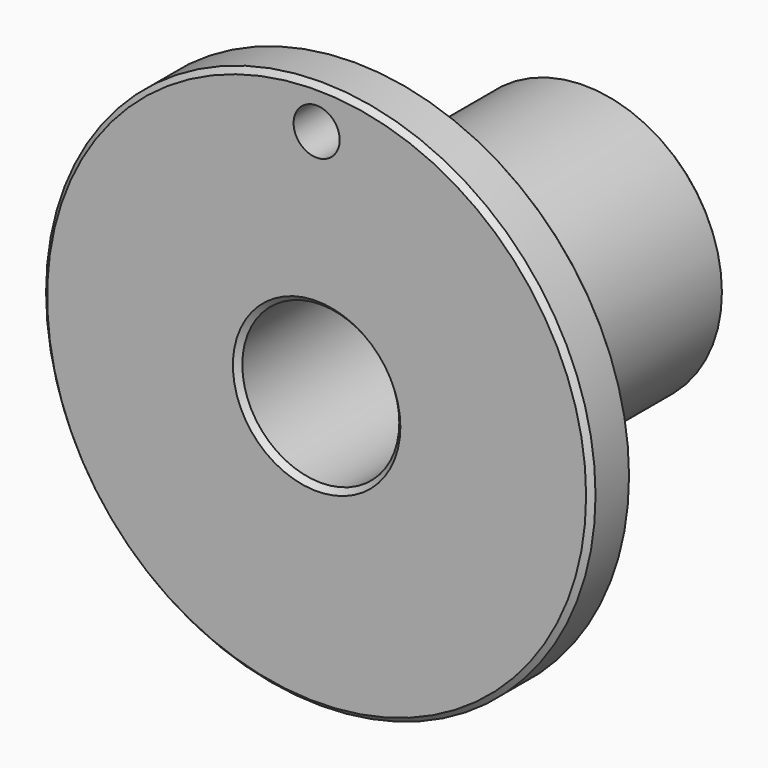
from build123d import *

# Parameters (mm, degrees)
F0_R         = 26.25
F1_DEPTH     = 55
F2_R         = 52.5
F2_R_2       = 26.25
F3_DEPTH     = 10
F6_D         = 30
F6_DEPTH     = 40
F6_TIP       = 9.0129092854
F7_D         = 40
F7_DEPTH     = 30
F7_TIP       = 12.0172123806
F8_T10_ANGLE = 180
F8_T12_ANGLE = 180
F10_D        = 8.8


# Not quite as in the source:
# - a fillet or chamfer that OpenCascade refuses, or shapes differently, is made with other operations: its cross-section is extruded or revolved along the edge and cut away or added


with BuildPart() as f1:
    # F0 (on Front) → F1 (new body)
    with BuildSketch(Plane.XZ):
        Circle(F0_R)
    extrude(amount=F1_DEPTH)

    # F2 (on face) → F3 (join)
    with BuildSketch(Plane.XZ.offset(55)):
        Circle(F2_R)
        Circle(F2_R_2, mode=Mode.SUBTRACT)
        Circle(F2_R_2)
    extrude(amount=F3_DEPTH)

    # F6
    with Locations(Plane.XZ.offset(65)):
        with Locations((0, 0)):
            Hole(F6_D / 2, depth=F6_DEPTH)
            with Locations((0, 0, -(F6_DEPTH + F6_TIP / 2))):  # 118° drill point
                Cone(0, F6_D / 2, F6_TIP, mode=Mode.SUBTRACT)

    # F7
    with Locations(Plane(origin=(0, 0, 0), x_dir=(-1, 0, 0), z_dir=(0, 1, 0))):
        with Locations((0, 0)):
            Hole(F7_D / 2, depth=F7_DEPTH)
            with Locations((0, 0, -(F7_DEPTH + F7_TIP / 2))):  # 118° drill point
                Cone(0, F7_D / 2, F7_TIP, mode=Mode.SUBTRACT)

    # F8: chamfer of 1 on 7 edges, made by hand

    # F8_s1 → F8_t2 (revolve, cut)
    with BuildSketch(Plane.XY):
        Polygon((52.5, -56), (51.5, -55), (52.5, -55), align=None)
    revolve(axis=Axis((0, -55, 0), (0, -1, 0)), mode=Mode.SUBTRACT)

    # F8_s3 → F8_t4 (revolve, cut)
    with BuildSketch(Plane.XY):
        Polygon((26.25, -1), (25.25, 0), (26.25, 0), align=None)
    revolve(axis=Axis((0, 0, 0), (0, -1, 0)), mode=Mode.SUBTRACT)

    # F8_s5 → F8_t6 (revolve, cut)
    with BuildSketch(Plane.XY):
        Polygon((52.5, -64), (51.5, -65), (52.5, -65), align=None)
    revolve(axis=Axis((0, -65, 0), (0, -1, 0)), mode=Mode.SUBTRACT)

    # F8_s7 → F8_t8 (revolve, cut)
    with BuildSketch(Plane.XY):
        Polygon((16, -65), (15, -64), (15, -65), align=None)
    revolve(axis=Axis((0, -65, 0), (0, -1, 0)), mode=Mode.SUBTRACT)

    # F8_s9 → F8_t10 (revolve, cut)
    with BuildSketch(Plane.XY):
        Polygon((-15, -33.5700758733), (-15.4849619251, -32.7129085726), (-15, -33.0043030951), align=None)
    revolve(axis=Axis((0, -33.0043030951, 0), (0, -1, 0)), revolution_arc=F8_T10_ANGLE, mode=Mode.SUBTRACT)

    # F8_s11 → F8_t12 (revolve, cut)
    with BuildSketch(Plane.XY):
        Polygon((15, -33.5700758733), (15.4849619251, -32.7129085726), (15, -33.0043030951), align=None)
    revolve(axis=Axis((0, -33.0043030951, 0), (0, -1, 0)), revolution_arc=F8_T12_ANGLE, mode=Mode.SUBTRACT)

    # F8_s13 → F8_t14 (revolve, cut)
    with BuildSketch(Plane.XY):
        Polygon((-21, 0), (-20, -1), (-20, 0), align=None)
    revolve(axis=Axis((0, 0, 0), (0, 1, 0)), mode=Mode.SUBTRACT)

    # F10 (through all)
    with Locations(Plane.XZ.offset(65)):
        with Locations((0, 44.5)):
            Hole(F10_D / 2)


solid = f1.part
